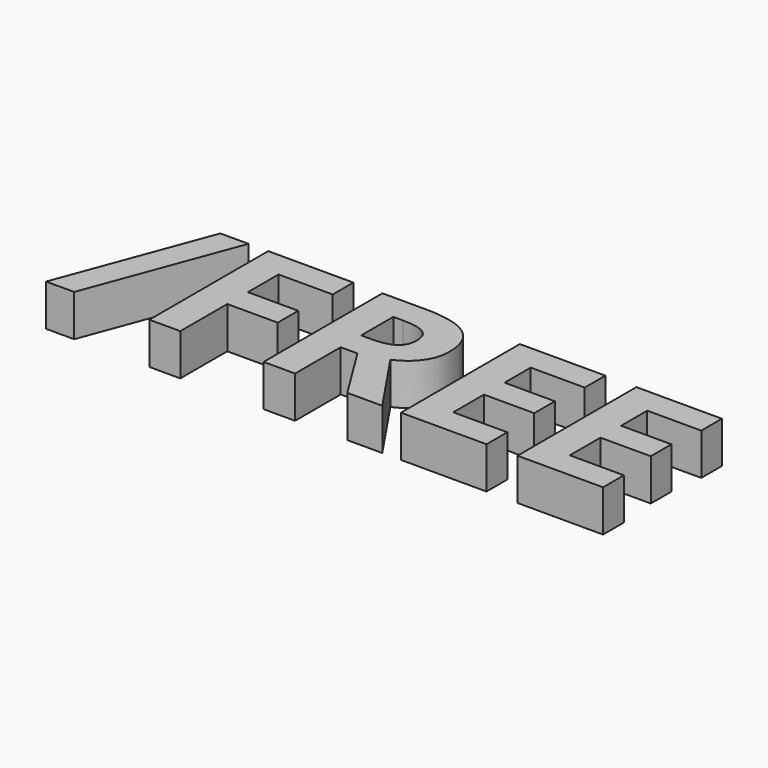
from build123d import *

# Parameters (mm, degrees)
F0_TEXT_SIZE = 25
F1_DEPTH     = 5


# Not quite as in the source:
# - Text() gives the source's letters only with a copy of the font that has no kerning and outlines rounded to 1/6400 em; it was checked with that copy


with BuildPart() as f1:
    # F0 (on Top) → F1 (new body)
    with BuildSketch(Plane.XY):
        with Locations((-14.8026317129, -9)):
            Text('/FREE', F0_TEXT_SIZE, font='Open Sans', font_style=FontStyle.BOLD, text_align=(TextAlign.LEFT, TextAlign.BOTTOM))
    extrude(amount=F1_DEPTH)


solid = f1.part
